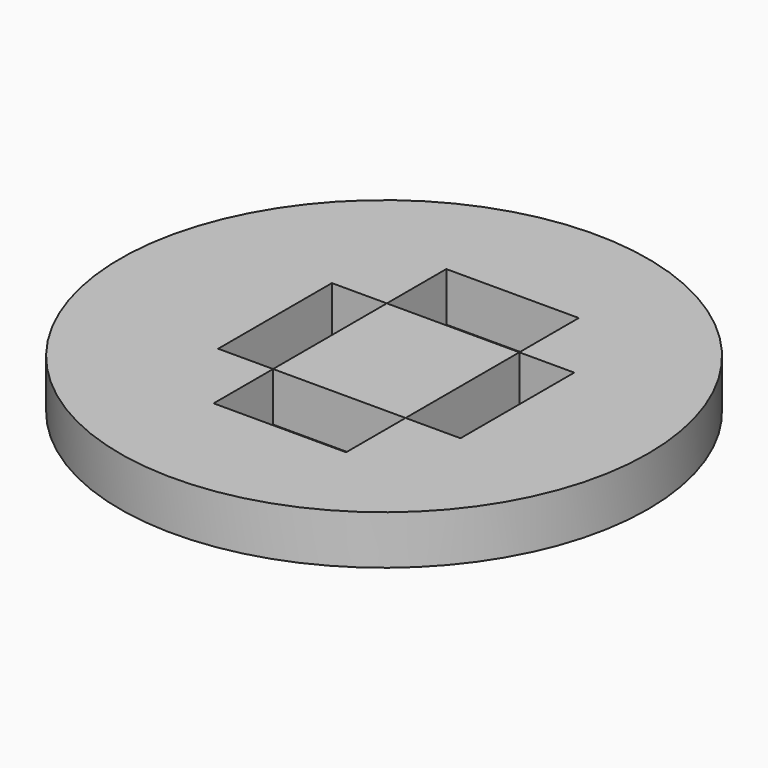
from build123d import *

# Parameters (mm, degrees)
F0_W     = 15.8282737248
F0_H     = 16.9864408672
F1_DEPTH = 5.842
F0_R     = 31.5328718462


# Not quite as in the source:
# - a feature of the source that left no trace in its solid (it failed there, or was rolled back) is left out


with BuildPart() as f1:
    # F0 (on Top) → F1 (new body)
    with BuildSketch(Plane.XY):
        with Locations((1.4477076475, 0)):
            Rectangle(F0_W, F0_H)
    extrude(amount=F1_DEPTH)


with BuildPart() as f1b:
    # F0 (on Top) → F1, piece 2 (new body)
    with BuildSketch(Plane.XY):
        Circle(F0_R)
        Polygon((9.3618445098, 8.4932204336), (15.9247908741, 8.4932204336), (15.9247908741, -8.4932204336), (9.3618445098, -8.4932204336), (9.3618445098, -17.3724964261), (-6.4664292149, -17.3724964261), (-6.4664292149, -8.4932204336), (-13.0293755792, -8.4932204336), (-13.0293755792, 8.4932204336), (-6.4664292149, 8.4932204336), (-6.4664292149, 17.3724964261), (9.3618445098, 17.3724964261), align=None, mode=Mode.SUBTRACT)
    extrude(amount=F1_DEPTH)


solid = Compound([f1.part, f1b.part])
